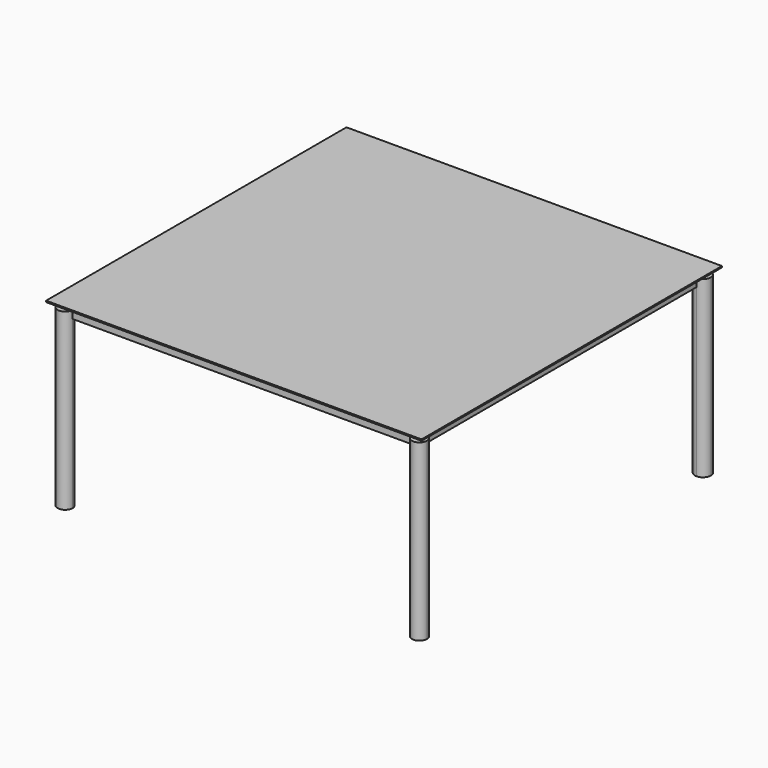
from build123d import *

# Parameters (mm, degrees)
F0_W      = 670
F0_H      = 670
F1_DEPTH  = 15
F2_W      = 650
F2_H      = 650
F3_DEPTH  = 15.001
F5_DEPTH  = 315
F6_DEPTH  = 15
F7_R      = 5
F8_DEPTH  = 10
F10_DEPTH = 315
F11_DEPTH = 15
F12_R     = 5
F13_DEPTH = 10
F15_DEPTH = 315
F16_DEPTH = 15
F17_R     = 5
F18_DEPTH = 10
F20_R     = 5
F21_DEPTH = 10
F22_DEPTH = 315
F23_DEPTH = 15
F24_W     = 710
F24_H     = 710
F24_R     = 5
F25_DEPTH = 2.5


with BuildPart() as f1:
    # F0 (on Top) → F1 (new body)
    with BuildSketch(Plane.XY):
        Rectangle(F0_W, F0_H)
    extrude(amount=F1_DEPTH)

    # F2 (on face) → F3 (cut, through all)
    with BuildSketch(Plane.XY.offset(15)):
        Rectangle(F2_W, F2_H)
    extrude(amount=-F3_DEPTH, mode=Mode.SUBTRACT)

    # F4 (on face) → F5 (join)
    with BuildSketch(Plane(origin=(0, 0, 0), x_dir=(1, 0, 0), z_dir=(0, 0, -1))):
        with BuildLine():
            Line((335, -335), (335, -320))
            ThreePointArc((335, -320), (329.647669, -320.987415), (325, -323.81966))
            Line((325, -323.81966), (325, -325))
            Line((325, -325), (323.81966, -325))
            ThreePointArc((323.81966, -325), (320.987415, -329.647669), (320, -335))
            Line((320, -335), (335, -335))
        make_face()
        with BuildLine():
            Line((325, -325), (325, -323.81966))
            ThreePointArc((325, -323.81966), (324.393398, -324.393398), (323.81966, -325))
            Line((323.81966, -325), (325, -325))
        make_face()
        with BuildLine():
            ThreePointArc((320, -335), (335, -350), (350, -335))
            ThreePointArc((350, -335), (345.606602, -324.393398), (335, -320))
            Line((335, -320), (335, -335))
            Line((335, -335), (320, -335))
        make_face()
    extrude(amount=F5_DEPTH)

    # F6 (add): a face of the model
    f6_faces = [f1.faces().sort_by_distance(p)[0] for p in [
        (337.122066, 337.122066, 0),
    ]]
    extrude(f6_faces, amount=F6_DEPTH)

    # F7 (on face) → F8 (join)
    with BuildSketch(Plane.XY.offset(15)):
        with Locations((335, 335)):
            Circle(F7_R)
    extrude(amount=F8_DEPTH)

    # F9 (on face) → F10 (join)
    with BuildSketch(Plane(origin=(0, 0, 0), x_dir=(1, 0, 0), z_dir=(0, 0, -1))):
        with BuildLine():
            ThreePointArc((-335, -320.857864), (-345, -345), (-320.857864, -335))
            Line((-320.857864, -335), (-335, -335))
            Line((-335, -335), (-335, -320.857864))
        make_face()
        with BuildLine():
            Line((-335, -335), (-320.857864, -335))
            ThreePointArc((-320.857864, -335), (-321.93437, -329.588039), (-325, -325))
            ThreePointArc((-325, -325), (-329.588039, -321.93437), (-335, -320.857864))
            Line((-335, -320.857864), (-335, -335))
        make_face()
    extrude(amount=F10_DEPTH)

    # F11 (add): a face of the model
    f11_faces = [f1.faces().sort_by_distance(p)[0] for p in [
        (-337.000703, 337.000703, 0),
    ]]
    extrude(f11_faces, amount=F11_DEPTH)

    # F12 (on face) → F13 (join)
    with BuildSketch(Plane.XY.offset(15)):
        with Locations((-335, 335)):
            Circle(F12_R)
    extrude(amount=F13_DEPTH)

    # F14 (on face) → F15 (join)
    with BuildSketch(Plane(origin=(0, 0, 0), x_dir=(1, 0, 0), z_dir=(0, 0, -1))):
        with BuildLine():
            Line((-335, 335), (-320.857864, 335))
            ThreePointArc((-320.857864, 335), (-345, 345), (-335, 320.857864))
            Line((-335, 320.857864), (-335, 335))
        make_face()
        with BuildLine():
            ThreePointArc((-335, 320.857864), (-329.588039, 321.93437), (-325, 325))
            ThreePointArc((-325, 325), (-321.93437, 329.588039), (-320.857864, 335))
            Line((-320.857864, 335), (-335, 335))
            Line((-335, 335), (-335, 320.857864))
        make_face()
    extrude(amount=F15_DEPTH)

    # F16 (add): a face of the model
    f16_faces = [f1.faces().sort_by_distance(p)[0] for p in [
        (-337.000703, -337.000703, 0),
    ]]
    extrude(f16_faces, amount=F16_DEPTH)

    # F17 (on face) → F18 (join)
    with BuildSketch(Plane.XY.offset(15)):
        with Locations((-335, -335)):
            Circle(F17_R)
    extrude(amount=F18_DEPTH)

    # F20 (on face) → F21 (join)
    with BuildSketch(Plane.XY.offset(15)):
        with Locations((335, -335)):
            Circle(F20_R)
    extrude(amount=F21_DEPTH)

    # F19 (on face) → F22 (join)
    with BuildSketch(Plane(origin=(0, 0, 0), x_dir=(1, 0, 0), z_dir=(0, 0, -1))):
        with BuildLine():
            ThreePointArc((335, 320.857864), (345, 325), (349.142136, 335))
            ThreePointArc((349.142136, 335), (335, 349.142136), (320.857864, 335))
            Line((320.857864, 335), (335, 335))
            Line((335, 335), (335, 320.857864))
        make_face()
        with BuildLine():
            Line((335, 335), (320.857864, 335))
            ThreePointArc((320.857864, 335), (321.93437, 329.588039), (325, 325))
            ThreePointArc((325, 325), (329.588039, 321.93437), (335, 320.857864))
            Line((335, 320.857864), (335, 335))
        make_face()
    extrude(amount=F22_DEPTH)

    # F23 (add): a face of the model
    f23_faces = [f1.faces().sort_by_distance(p)[0] for p in [
        (337.000703, -337.000703, 0),
    ]]
    extrude(f23_faces, amount=F23_DEPTH)

    # F24 (on face) → F25 (join)
    with BuildSketch(Plane.XY.offset(25)):
        Rectangle(F24_W, F24_H)
        with Locations((-335, 335)):
            Circle(F24_R, mode=Mode.SUBTRACT)
        with Locations((-335, 335)):
            Circle(F24_R)
    extrude(amount=F25_DEPTH)


solid = f1.part
